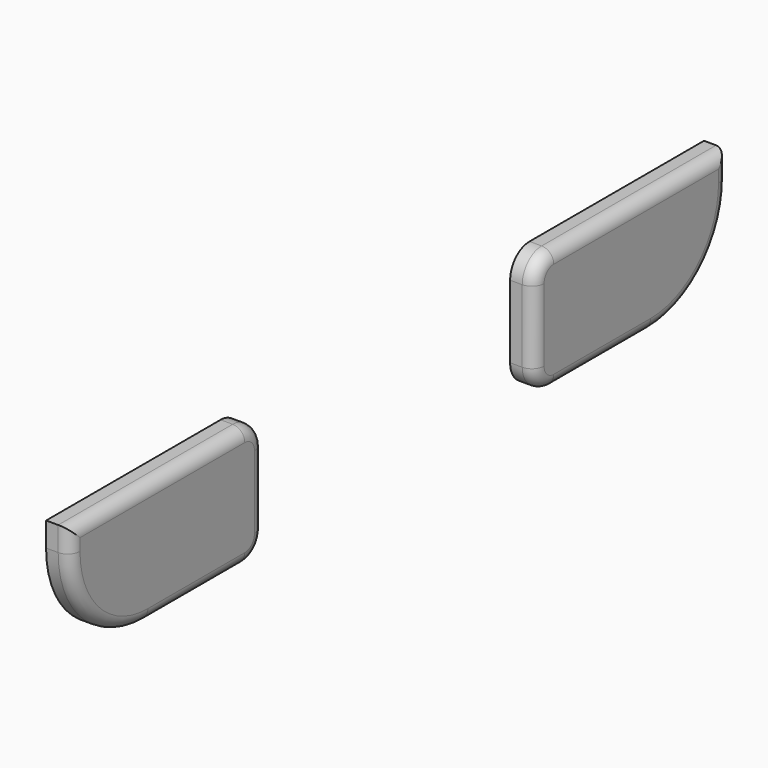
from build123d import *

# Parameters (mm, degrees)
F0_W        = 12.7
F0_H        = 6.35
F1_DEPTH    = 1.27
F2_R        = 0.635
F2_2_R      = 0.635
F3_T1_DEPTH = 13.97
F3_T4_ANGLE = 90
F4_T1_DEPTH = 13.97
F4_T4_ANGLE = 90
F5_T1_DEPTH = 4.445
F5_T4_ANGLE = 90
F6_T1_DEPTH = 4.445
F6_T4_ANGLE = 90
F7_T1_DEPTH = 4.445
F7_T4_ANGLE = 90
F8_T1_DEPTH = 4.445
F8_T4_ANGLE = 90


# Not quite as in the source:
# - a fillet or chamfer that OpenCascade refuses, or shapes differently, is made with other operations: its cross-section is extruded or revolved along the edge and cut away or added


with BuildPart() as f1:
    # F0 (on Right) → F1 (new body)
    with BuildSketch(Plane.YZ):
        with Locations((-31.4221102744, 33.8466549292)):
            Rectangle(F0_W, F0_H)
    extrude(amount=F1_DEPTH)

    # F2
    f2_edges = [f1.edges().sort_by_distance(p)[0] for p in [
        (1.27, -31.42211, 37.021655),
        (1.27, -25.07211, 33.846655),
        (1.27, -31.42211, 30.671655),
        (1.27, -37.77211, 33.846655),
    ]]
    fillet(f2_edges, radius=F2_R)

    # F4: fillet of radius 5.08 on 1 edges, made by hand

    # F4_s2 → F4_t1 (cut)
    with BuildSketch(Plane.YZ.offset(-12.7)):
        with BuildLine():
            ThreePointArc((-37.7721102744, 35.7516549292), (-36.2842127229, 32.1595524808), (-32.6921102744, 30.6716549292))
            Line((-32.6921102744, 30.6716549292), (-37.7721102744, 30.6716549292))
            Line((-37.7721102744, 30.6716549292), (-37.7721102744, 35.7516549292))
        make_face()
    extrude(amount=F4_T1_DEPTH, mode=Mode.SUBTRACT)

    # F4_s3 → F4_t4 (revolve, cut)
    with BuildSketch(Plane.XY.offset(35.7516549292)):
        with BuildLine():
            ThreePointArc((1.27, -37.1371102744), (1.0840128061, -37.5861230805), (0.635, -37.7721102744))
            Line((0.635, -37.7721102744), (1.27, -37.7721102744))
            Line((1.27, -37.7721102744), (1.27, -37.1371102744))
        make_face()
    revolve(axis=Axis((1.27, -32.6921102744, 35.7516549292), (1, 0, 0)), revolution_arc=F4_T4_ANGLE, mode=Mode.SUBTRACT)

    # F5: fillet of radius 1.27 on 1 edges, made by hand

    # F5_s2 → F5_t1 (cut)
    with BuildSketch(Plane.YZ.offset(-3.175)):
        with BuildLine():
            ThreePointArc((-26.3421102744, 37.0216549292), (-25.4440846623, 36.6496805413), (-25.0721102744, 35.7516549292))
            Line((-25.0721102744, 35.7516549292), (-25.0721102744, 37.0216549292))
            Line((-25.0721102744, 37.0216549292), (-26.3421102744, 37.0216549292))
        make_face()
    extrude(amount=F5_T1_DEPTH, mode=Mode.SUBTRACT)

    # F5_s3 → F5_t4 (revolve, cut)
    with BuildSketch(Plane.XY.offset(35.7516549292)):
        with BuildLine():
            ThreePointArc((1.27, -25.7071102744), (1.0840128061, -25.2580974684), (0.635, -25.0721102744))
            Line((0.635, -25.0721102744), (1.27, -25.0721102744))
            Line((1.27, -25.0721102744), (1.27, -25.7071102744))
        make_face()
    revolve(axis=Axis((1.27, -26.3421102744, 35.7516549292), (1, 0, 0)), revolution_arc=F5_T4_ANGLE, mode=Mode.SUBTRACT)

    # F7: fillet of radius 1.27 on 1 edges, made by hand

    # F7_s2 → F7_t1 (cut)
    with BuildSketch(Plane.YZ.offset(-3.175)):
        with BuildLine():
            ThreePointArc((-25.0721102744, 31.9416549292), (-25.4440846623, 31.0436293171), (-26.3421102744, 30.6716549292))
            Line((-26.3421102744, 30.6716549292), (-25.0721102744, 30.6716549292))
            Line((-25.0721102744, 30.6716549292), (-25.0721102744, 31.9416549292))
        make_face()
    extrude(amount=F7_T1_DEPTH, mode=Mode.SUBTRACT)

    # F7_s3 → F7_t4 (revolve, cut)
    with BuildSketch(Plane.XZ.offset(26.3421102744)):
        with BuildLine():
            ThreePointArc((1.27, 31.3066549292), (1.0840128061, 30.8576421232), (0.635, 30.6716549292))
            Line((0.635, 30.6716549292), (1.27, 30.6716549292))
            Line((1.27, 30.6716549292), (1.27, 31.3066549292))
        make_face()
    revolve(axis=Axis((1.27, -26.3421102744, 31.9416549292), (1, 0, 0)), revolution_arc=F7_T4_ANGLE, mode=Mode.SUBTRACT)


with BuildPart() as f1b:
    # F0 (on Right) → F1, piece 2 (new body)
    with BuildSketch(Plane.YZ):
        with Locations((-1.0206177063, 33.8466549292)):
            Rectangle(F0_W, F0_H)
    extrude(amount=F1_DEPTH)

    # F2#2
    f2_2_edges = [f1b.edges().sort_by_distance(p)[0] for p in [
        (1.27, -1.020618, 37.021655),
        (1.27, -7.370618, 33.846655),
        (1.27, -1.020618, 30.671655),
        (1.27, 5.329382, 33.846655),
    ]]
    fillet(f2_2_edges, radius=F2_2_R)

    # F3: fillet of radius 5.08 on 1 edges, made by hand

    # F3_s2 → F3_t1 (cut)
    with BuildSketch(Plane.YZ.offset(-12.7)):
        with BuildLine():
            ThreePointArc((5.3293822937, 35.7516549292), (3.8414847421, 32.1595524808), (0.2493822937, 30.6716549292))
            Line((0.2493822937, 30.6716549292), (5.3293822937, 30.6716549292))
            Line((5.3293822937, 30.6716549292), (5.3293822937, 35.7516549292))
        make_face()
    extrude(amount=F3_T1_DEPTH, mode=Mode.SUBTRACT)

    # F3_s3 → F3_t4 (revolve, cut)
    with BuildSketch(Plane.XZ.offset(-0.2493822937)):
        with BuildLine():
            ThreePointArc((1.27, 31.3066549292), (1.0840128061, 30.8576421232), (0.635, 30.6716549292))
            Line((0.635, 30.6716549292), (1.27, 30.6716549292))
            Line((1.27, 30.6716549292), (1.27, 31.3066549292))
        make_face()
    revolve(axis=Axis((1.27, 0.2493822937, 35.7516549292), (1, 0, 0)), revolution_arc=F3_T4_ANGLE, mode=Mode.SUBTRACT)

    # F6: fillet of radius 1.27 on 1 edges, made by hand

    # F6_s2 → F6_t1 (cut)
    with BuildSketch(Plane.YZ.offset(-3.175)):
        with BuildLine():
            ThreePointArc((-6.1006177063, 37.0216549292), (-6.9986433184, 36.6496805413), (-7.3706177063, 35.7516549292))
            Line((-7.3706177063, 35.7516549292), (-7.3706177063, 37.0216549292))
            Line((-7.3706177063, 37.0216549292), (-6.1006177063, 37.0216549292))
        make_face()
    extrude(amount=F6_T1_DEPTH, mode=Mode.SUBTRACT)

    # F6_s3 → F6_t4 (revolve, cut)
    with BuildSketch(Plane.XZ.offset(6.1006177063)):
        with BuildLine():
            ThreePointArc((1.27, 36.3866549292), (1.0840128061, 36.8356677353), (0.635, 37.0216549292))
            Line((0.635, 37.0216549292), (1.27, 37.0216549292))
            Line((1.27, 37.0216549292), (1.27, 36.3866549292))
        make_face()
    revolve(axis=Axis((1.27, -6.1006177063, 35.7516549292), (1, 0, 0)), revolution_arc=F6_T4_ANGLE, mode=Mode.SUBTRACT)

    # F8: fillet of radius 1.27 on 1 edges, made by hand

    # F8_s2 → F8_t1 (cut)
    with BuildSketch(Plane.YZ.offset(-3.175)):
        with BuildLine():
            ThreePointArc((-6.1006177063, 30.6716549292), (-6.9986433184, 31.0436293171), (-7.3706177063, 31.9416549292))
            Line((-7.3706177063, 31.9416549292), (-7.3706177063, 30.6716549292))
            Line((-7.3706177063, 30.6716549292), (-6.1006177063, 30.6716549292))
        make_face()
    extrude(amount=F8_T1_DEPTH, mode=Mode.SUBTRACT)

    # F8_s3 → F8_t4 (revolve, cut)
    with BuildSketch(Plane.XY.offset(31.9416549292)):
        with BuildLine():
            ThreePointArc((1.27, -6.7356177063), (1.0840128061, -7.1846305124), (0.635, -7.3706177063))
            Line((0.635, -7.3706177063), (1.27, -7.3706177063))
            Line((1.27, -7.3706177063), (1.27, -6.7356177063))
        make_face()
    revolve(axis=Axis((1.27, -6.1006177063, 31.9416549292), (1, 0, 0)), revolution_arc=F8_T4_ANGLE, mode=Mode.SUBTRACT)


solid = Compound([f1.part, f1b.part])
